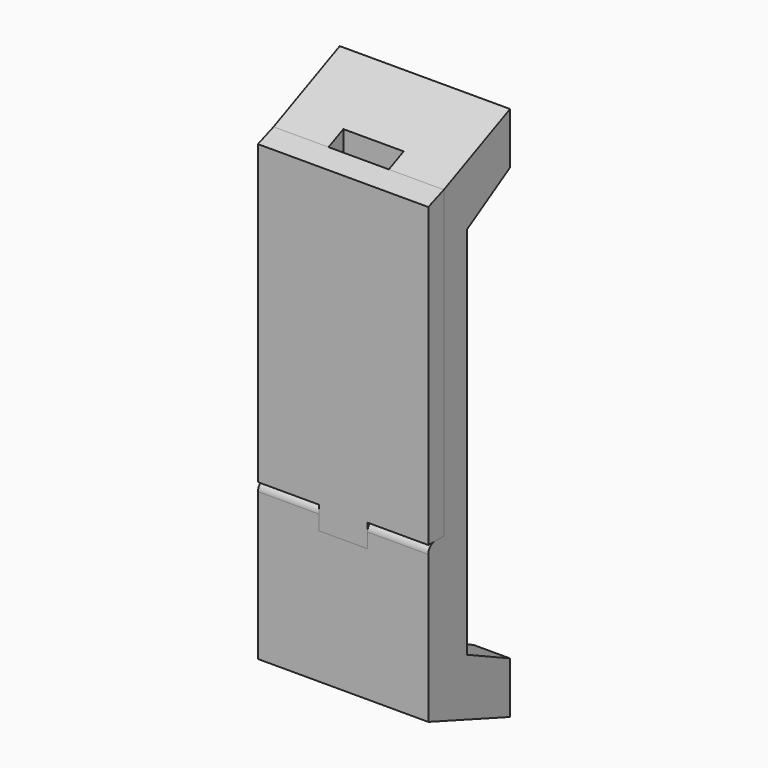
from build123d import *

# Parameters (mm, degrees)
F0_W      = 350
F0_H      = 674
F1_DEPTH  = 40
F2_W      = 344
F2_H      = 586.6
F3_DEPTH  = 36
F4_W      = 310
F4_H      = 50
F4_W_2    = 300
F4_H_2    = 40
F5_DEPTH  = 37
F6_R      = 5
F7_DEPTH  = 150
F8_W      = 125
F8_H      = 80.1298069
F8_H_2    = 76.0073708534
F9_DEPTH  = 40.001
F10_R     = 20
F11_R     = 5
F12_DEPTH = 25
F13_R     = 5
F14_DEPTH = 25
F16_DEPTH = 350.001
F17_W     = 80
F17_H     = 79.4738833577
F18_DEPTH = 36
F20_DEPTH = 175
F22_DEPTH = 38
F24_DEPTH = 38
F26_DEPTH = 100
F27_W     = 40
F27_H     = 52.4
F28_DEPTH = 50
F30_DEPTH = 170
F31_W     = 115
F31_H     = 42.4
F32_DEPTH = 40
F33_R     = 5
F34_DEPTH = 5
F35_R     = 5
F36_DEPTH = 5
F37_R     = 17


with BuildPart() as f1:
    # F0 (on Front) → F1 (new body)
    with BuildSketch(Plane.XZ):
        with Locations((0, 27)):
            Rectangle(F0_W, F0_H)
    extrude(amount=F1_DEPTH)

    # F2 (on face) → F3 (cut)
    with BuildSketch(Plane(origin=(0, 0, 0), x_dir=(-1, 0, 0), z_dir=(0, 1, 0))):
        with Locations((0, 55.7)):
            Rectangle(F2_W, F2_H)
    extrude(amount=-F3_DEPTH, mode=Mode.SUBTRACT)

    # F4 (on face) → F5 (join)
    with BuildSketch(Plane(origin=(0, -36, 0), x_dir=(-1, 0, 0), z_dir=(0, 1, 0))):
        with Locations((0, 47.4)):
            Rectangle(F4_W, F4_H)
        with Locations((0, 47.4)):
            Rectangle(F4_W_2, F4_H_2, mode=Mode.SUBTRACT)
    extrude(amount=F5_DEPTH)

    # F6 (on Right) → F7 (join, symmetric)
    with BuildSketch(Plane.YZ):
        with Locations((-4, 47.4)):
            Circle(F6_R)
    extrude(amount=F7_DEPTH, both=True)

    # F8 (on face) → F9 (cut, through all)
    with BuildSketch(Plane(origin=(0, 0, 0), x_dir=(-1, 0, 0), z_dir=(0, 1, 0))):
        with Locations((-112.5, -302.66490345)):
            Rectangle(F8_W, F8_H)
        with Locations((112.5, -300.6036854267)):
            Rectangle(F8_W, F8_H_2)
    extrude(amount=-F9_DEPTH, mode=Mode.SUBTRACT)

    # F10
    f10_edges = [f1.edges().sort_by_distance(p)[0] for p in [
        (0, 0, -310),
    ]]
    fillet(f10_edges, radius=F10_R)

    # F11 (on face) → F12 (join)
    with BuildSketch(Plane.YZ.offset(50)):
        with Locations((-20, -300)):
            Circle(F11_R)
    extrude(amount=F12_DEPTH)

    # F13 (on face) → F14 (join)
    with BuildSketch(Plane(origin=(-50, 0, 0), x_dir=(0, -1, 0), z_dir=(-1, 0, 0))):
        with Locations((20, -300)):
            Circle(F13_R)
    extrude(amount=F14_DEPTH)

    # F15 (on face) → F16 (cut, through all)
    with BuildSketch(Plane(origin=(-175, 0, 0), x_dir=(0, -1, 0), z_dir=(-1, 0, 0))):
        Polygon((40, 364), (0, 364), (40, 349), align=None)
    extrude(amount=-F16_DEPTH, mode=Mode.SUBTRACT)

    # F17 (on face) → F18 (cut, through all)
    with BuildSketch(Plane(origin=(0, 0, 0), x_dir=(-1, 0, 0), z_dir=(0, 1, 0))):
        with Locations((0, -235.2630583211)):
            Rectangle(F17_W, F17_H)
    extrude(amount=-F18_DEPTH, mode=Mode.SUBTRACT)


with BuildPart() as f20:
    # F19 (on Right) → F20 (new body, symmetric)
    with BuildSketch(Plane.YZ):
        Polygon((-40, -582.6), (170, -659.0337491959), (170, -553.0337491959), (60, -501.7399067989), (60, 268.2600932011), (170, 334.9662508041), (170, 440.9662508041), (0, 364), (0, -262.6), (-40, -262.6), align=None)
    extrude(amount=F20_DEPTH, both=True)

    # F21 (on face) → F22 (cut)
    with BuildSketch(Plane.XZ):
        with BuildLine():
            Line((-72, 344), (-172, 344))
            Line((-172, 344), (-172, -257.6))
            Line((-172, -257.6), (172, -257.6))
            Line((172, -257.6), (172, 344))
            Line((172, 344), (72, 344))
            ThreePointArc((72, 344), (0, 272), (-72, 344))
        make_face()
    extrude(amount=-F22_DEPTH, mode=Mode.SUBTRACT)

    # F23 (on face) → F24 (cut)
    with BuildSketch(Plane.XZ):
        with BuildLine():
            Line((-62, 388.1143927574), (-62, 344))
            ThreePointArc((-62, 344), (0, 282), (62, 344))
            Line((62, 344), (62, 388.1143927574))
            Line((62, 388.1143927574), (-62, 388.1143927574))
        make_face()
    extrude(amount=-F24_DEPTH, mode=Mode.SUBTRACT)

    # F25 (on Right) → F26 (cut, symmetric)
    with BuildSketch(Plane.YZ):
        Polygon((170, -633.0337491959), (170, -553.0337491959), (170, -466.1389887333), (60, -501.7399067989), (60, -592.9970234266), align=None)
        Polygon((170, 334.9662508041), (170, 414.9662508041), (60, 368.399853225), (60, 268.2600932011), (170, 214.6935015917), align=None)
    extrude(amount=F26_DEPTH, both=True, mode=Mode.SUBTRACT)

    # F27 (on Right) → F28 (cut, symmetric)
    with BuildSketch(Plane.YZ):
        with Locations((-20, -283.8)):
            Rectangle(F27_W, F27_H)
    extrude(amount=F28_DEPTH, both=True, mode=Mode.SUBTRACT)

    # F29 (on Right) → F30 (cut, symmetric)
    with BuildSketch(Plane.YZ):
        Polygon((81.2916728854, -267.6), (5, -267.6), (5, -315), (-35, -315), (-35, -462.4406792741), (60, -501.7399067989), (81.2916728854, -331.8917108536), align=None)
    extrude(amount=F30_DEPTH, both=True, mode=Mode.SUBTRACT)

    # F31 (on face) → F32 (cut, through all)
    with BuildSketch(Plane(origin=(0, 5, 0), x_dir=(-1, 0, 0), z_dir=(0, 1, 0))):
        with Locations((-112.5, -293.8)):
            Rectangle(F31_W, F31_H)
        with Locations((112.5, -293.8)):
            Rectangle(F31_W, F31_H)
    extrude(amount=-F32_DEPTH, mode=Mode.SUBTRACT)

    # F33 (on face) → F34 (cut)
    with BuildSketch(Plane.YZ.offset(55)):
        with Locations((-20, -300)):
            Circle(F33_R)
    extrude(amount=-F34_DEPTH, mode=Mode.SUBTRACT)

    # F35 (on face) → F36 (cut)
    with BuildSketch(Plane(origin=(-55, 0, 0), x_dir=(0, -1, 0), z_dir=(-1, 0, 0))):
        with Locations((20, -300)):
            Circle(F35_R)
    extrude(amount=-F36_DEPTH, mode=Mode.SUBTRACT)

    # F37
    f37_edges = [f20.edges().sort_by_distance(p)[0] for p in [
        (-112.5, -40, -262.6),
        (112.5, -40, -262.6),
    ]]
    fillet(f37_edges, radius=F37_R)


solid = Compound([f1.part, f20.part])
